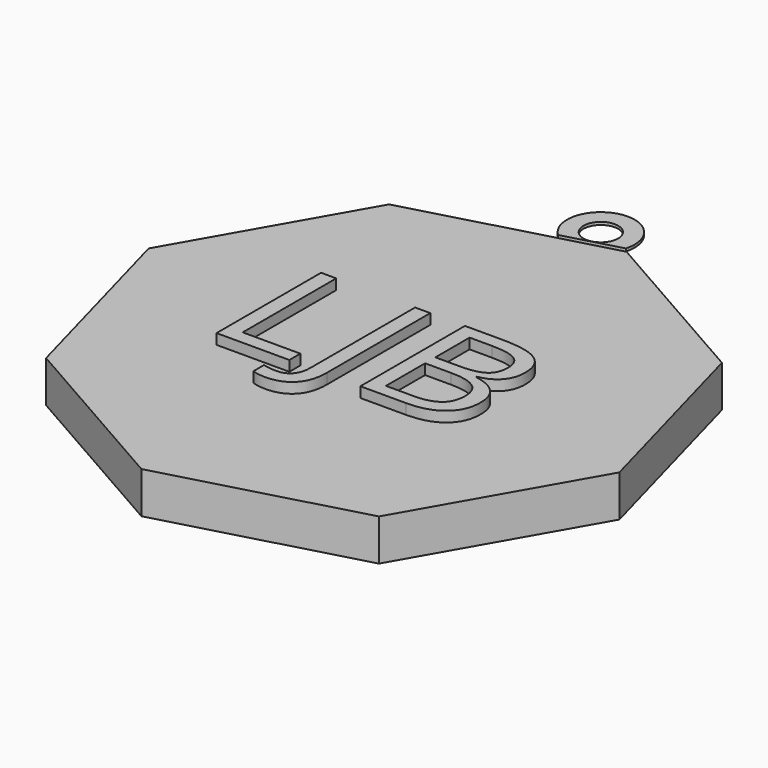
from build123d import *

# Parameters (mm, degrees)
F1_DEPTH     = 7.62
F2_TEXT_SIZE = 33.5773388441
F4_DEPTH     = 1.905
F7_DEPTH     = 0.508
F8_D         = 6.35


# Not quite as in the source:
# - Text() gives the source's letters only with a copy of the font that has no kerning and outlines rounded to 1/6400 em; it was checked with that copy


with BuildPart() as f1:
    # F0 (on Top) → F1 (new body)
    with BuildSketch(Plane.XY):
        Polygon((-38.2548050288, -29.674370654), (-6.067283332, -48.0331807657), (29.674370654, -38.2548050288), (48.0331807657, -6.067283332), (38.2548050288, 29.674370654), (6.067283332, 48.0331807657), (-29.674370654, 38.2548050288), (-48.0331807657, 6.067283332), align=None)
    extrude(amount=F1_DEPTH)

    # F2 (on face) → F4 (join)
    with BuildSketch(Plane.XY.offset(7.62)):
        with Locations((-25.0391010195, -11.2244244665)):
            Text('LJB', F2_TEXT_SIZE, font='Open Sans', text_align=(TextAlign.LEFT, TextAlign.BOTTOM))
    extrude(amount=F4_DEPTH)


with BuildPart() as f7:
    # F5 (on face) → F7 (new body)
    with BuildSketch(Plane.XY.offset(7.62)):
        with BuildLine():
            ThreePointArc((5.952275919, 48.0017164777), (6.1364816563, 48.8574833632), (6.1982945238, 49.7306659818))
            ThreePointArc((6.1982945238, 49.7306659818), (-2.461570663, 55.4192092816), (-4.2431340822, 45.2124065643))
            Line((-4.2431340822, 45.2124065643), (5.952275919, 48.0017164777))
        make_face()
    extrude(amount=F7_DEPTH)

    # F8 (through all)
    with Locations(Plane(origin=(0, 0, 7.62), x_dir=(1, 0, 0), z_dir=(0, 0, -1))):
        with Locations((0, -49.7306659818)):
            Hole(F8_D / 2)


solid = Compound([f1.part, f7.part])
